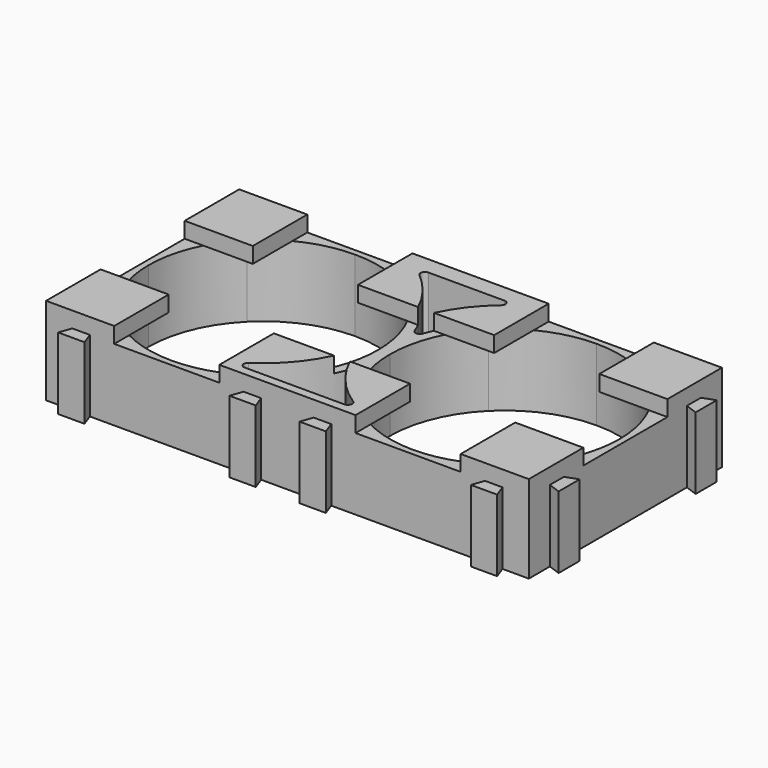
from build123d import *

# Parameters (mm, degrees)
F1_DEPTH = 8.2
F3_DEPTH = 1.8
F5_DEPTH = 8


# Not quite as in the source:
# - a feature names something its author has since deleted; it is built from what else it names


with BuildPart() as f1:
    # F0 (on Top) → F1 (new body)
    with BuildSketch(Plane.XY):
        with BuildLine():
            Line((13.775, 10.775), (13.775, 13.775))
            Line((13.775, 13.775), (10.775, 13.775))
            Line((10.775, 13.775), (11.275, 12.375))
            Line((11.275, 12.375), (8.275, 12.375))
            Line((8.275, 12.375), (8.775, 13.775))
            Line((8.775, 13.775), (0, 13.775))
            Line((0, 13.775), (0, 13.1))
            ThreePointArc((0, 13.1), (9.2630988335, 9.2630988335), (13.1, 0))
            Line((13.1, 0), (13.775, 0))
            Line((13.775, 0), (13.775, 8.775))
            Line((13.775, 8.775), (13.775, 10.775))
        make_face()
        Polygon((15.175, 11.275), (13.775, 10.775), (13.775, 8.775), (15.175, 8.275), align=None)
        Polygon((15.175, -8.275), (13.775, -8.775), (13.775, -10.775), (15.175, -11.275), align=None)
        with BuildLine():
            Line((13.775, -8.775), (13.775, 0))
            Line((13.775, 0), (13.1, 0))
            ThreePointArc((13.1, 0), (12.1028218759, -5.013152964), (9.2630988335, -9.2630988335))
            Line((9.2630988335, -9.2630988335), (13.775, -13.775))
            Line((13.775, -13.775), (13.775, -10.775))
            Line((13.775, -10.775), (13.775, -8.775))
        make_face()
        with BuildLine():
            Line((13.775, -13.775), (9.2630988335, -9.2630988335))
            ThreePointArc((9.2630988335, -9.2630988335), (5.013152964, -12.1028218759), (0, -13.1))
            Line((0, -13.1), (0, -13.775))
            Line((0, -13.775), (8.775, -13.775))
            Line((8.775, -13.775), (10.775, -13.775))
            Line((10.775, -13.775), (13.775, -13.775))
        make_face()
        Polygon((11.275, -15.175), (10.775, -13.775), (8.775, -13.775), (8.275, -15.175), align=None)
        with BuildLine():
            ThreePointArc((0, -13.1), (-9.2630988335, -9.2630988335), (-13.1, 0))
            Line((-13.1, 0), (-13.775, 0))
            Line((-13.775, 0), (-13.775, -8.775))
            Line((-13.775, -8.775), (-12.375, -8.275))
            Line((-12.375, -8.275), (-12.375, -11.275))
            Line((-12.375, -11.275), (-13.775, -10.775))
            Line((-13.775, -10.775), (-13.775, -13.775))
            Line((-13.775, -13.775), (-10.775, -13.775))
            Line((-10.775, -13.775), (-8.775, -13.775))
            Line((-8.775, -13.775), (0, -13.775))
            Line((0, -13.775), (0, -13.1))
        make_face()
        Polygon((-8.275, -15.175), (-8.775, -13.775), (-10.775, -13.775), (-11.275, -15.175), align=None)
        with BuildLine():
            ThreePointArc((-13.1, 0), (-12.1028218759, 5.013152964), (-9.2630988335, 9.2630988335))
            Line((-9.2630988335, 9.2630988335), (-13.775, 13.775))
            Line((-13.775, 13.775), (-13.775, 10.775))
            Line((-13.775, 10.775), (-12.375, 11.275))
            Line((-12.375, 11.275), (-12.375, 8.275))
            Line((-12.375, 8.275), (-13.775, 8.775))
            Line((-13.775, 8.775), (-13.775, 0))
            Line((-13.775, 0), (-13.1, 0))
        make_face()
        with BuildLine():
            Line((0, 13.1), (0, 13.775))
            Line((0, 13.775), (-8.775, 13.775))
            Line((-8.775, 13.775), (-8.275, 12.375))
            Line((-8.275, 12.375), (-9.775, 12.375))
            Line((-9.775, 12.375), (-11.275, 12.375))
            Line((-11.275, 12.375), (-10.775, 13.775))
            Line((-10.775, 13.775), (-13.775, 13.775))
            Line((-13.775, 13.775), (-9.2630988335, 9.2630988335))
            ThreePointArc((-9.2630988335, 9.2630988335), (-5.013152964, 12.1028218759), (0, 13.1))
        make_face()
        with BuildLine():
            ThreePointArc((27.55, -13.1), (18.2869011665, -9.2630988335), (14.45, 0))
            Line((14.45, 0), (13.775, 0))
            Line((13.775, 0), (13.775, -8.775))
            Line((13.775, -8.775), (15.175, -8.275))
            Line((15.175, -8.275), (15.175, -11.275))
            Line((15.175, -11.275), (13.775, -10.775))
            Line((13.775, -10.775), (13.775, -13.775))
            Line((13.775, -13.775), (16.775, -13.775))
            Line((16.775, -13.775), (18.775, -13.775))
            Line((18.775, -13.775), (27.55, -13.775))
            Line((27.55, -13.775), (27.55, -13.1))
        make_face()
        with BuildLine():
            Line((18.2869011665, 9.2630988335), (13.775, 13.775))
            Line((13.775, 13.775), (13.775, 10.775))
            Line((13.775, 10.775), (15.175, 11.275))
            Line((15.175, 11.275), (15.175, 8.275))
            Line((15.175, 8.275), (13.775, 8.775))
            Line((13.775, 8.775), (13.775, 0))
            Line((13.775, 0), (14.45, 0))
            ThreePointArc((14.45, 0), (15.4471781241, 5.013152964), (18.2869011665, 9.2630988335))
        make_face()
        with BuildLine():
            Line((16.775, 13.775), (13.775, 13.775))
            Line((13.775, 13.775), (18.2869011665, 9.2630988335))
            ThreePointArc((18.2869011665, 9.2630988335), (22.536847036, 12.1028218759), (27.55, 13.1))
            Line((27.55, 13.1), (27.55, 13.775))
            Line((27.55, 13.775), (18.775, 13.775))
            Line((18.775, 13.775), (19.275, 12.375))
            Line((19.275, 12.375), (17.775, 12.375))
            Line((17.775, 12.375), (16.275, 12.375))
            Line((16.275, 12.375), (16.775, 13.775))
        make_face()
        with BuildLine():
            Line((27.55, 13.775), (27.55, 13.1))
            ThreePointArc((27.55, 13.1), (36.8130988335, 9.2630988335), (40.65, 0))
            Line((40.65, 0), (41.325, 0))
            Line((41.325, 0), (41.325, 8.775))
            Line((41.325, 8.775), (41.325, 10.775))
            Line((41.325, 10.775), (41.325, 13.775))
            Line((41.325, 13.775), (38.325, 13.775))
            Line((38.325, 13.775), (38.825, 12.375))
            Line((38.825, 12.375), (35.825, 12.375))
            Line((35.825, 12.375), (36.325, 13.775))
            Line((36.325, 13.775), (27.55, 13.775))
        make_face()
        Polygon((41.325, 10.775), (41.325, 8.775), (42.725, 8.275), (42.725, 11.275), align=None)
        Polygon((19.275, -15.175), (18.775, -13.775), (16.775, -13.775), (16.275, -15.175), align=None)
        Polygon((38.325, -13.775), (36.325, -13.775), (35.825, -15.175), (38.825, -15.175), align=None)
        Polygon((42.725, -8.275), (41.325, -8.775), (41.325, -10.775), (42.725, -11.275), align=None)
        with BuildLine():
            Line((41.325, 0), (40.65, 0))
            ThreePointArc((40.65, 0), (39.6528218759, -5.013152964), (36.8130988335, -9.2630988335))
            Line((36.8130988335, -9.2630988335), (41.325, -13.775))
            Line((41.325, -13.775), (41.325, -10.775))
            Line((41.325, -10.775), (41.325, -8.775))
            Line((41.325, -8.775), (41.325, 0))
        make_face()
        with BuildLine():
            ThreePointArc((36.8130988335, -9.2630988335), (32.563152964, -12.1028218759), (27.55, -13.1))
            Line((27.55, -13.1), (27.55, -13.775))
            Line((27.55, -13.775), (36.325, -13.775))
            Line((36.325, -13.775), (38.325, -13.775))
            Line((38.325, -13.775), (41.325, -13.775))
            Line((41.325, -13.775), (36.8130988335, -9.2630988335))
        make_face()
    extrude(amount=F1_DEPTH)

    # F2 (on face) → F3 (join)
    with BuildSketch(Plane.XY.offset(8.2)):
        Polygon((11.275, 12.375), (10.775, 13.775), (8.775, 13.775), (8.275, 12.375), align=None)
        Polygon((-8.775, 13.775), (-10.775, 13.775), (-11.275, 12.375), (-8.275, 12.375), align=None)
        Polygon((-12.375, 11.275), (-13.775, 10.775), (-13.775, 8.775), (-12.375, 8.275), align=None)
        Polygon((-13.775, -8.775), (-13.775, -10.775), (-12.375, -11.275), (-12.375, -8.275), align=None)
        Polygon((18.775, 13.775), (16.775, 13.775), (16.275, 12.375), (19.275, 12.375), align=None)
        Polygon((38.325, 13.775), (36.325, 13.775), (35.825, 12.375), (38.825, 12.375), align=None)
        with BuildLine():
            ThreePointArc((21.55, 11.6451706729), (18.2869011665, 9.2630988335), (15.9048293271, 6))
            Line((15.9048293271, 6), (21.55, 6))
            Line((21.55, 6), (21.55, 11.6451706729))
        make_face()
        with BuildLine():
            ThreePointArc((39.1951706729, 6), (36.8130988335, 9.2630988335), (33.55, 11.6451706729))
            Line((33.55, 11.6451706729), (33.55, 6))
            Line((33.55, 6), (39.1951706729, 6))
        make_face()
        with BuildLine():
            Line((33.55, -6), (33.55, -11.6451706729))
            ThreePointArc((33.55, -11.6451706729), (36.8130988335, -9.2630988335), (39.1951706729, -6))
            Line((39.1951706729, -6), (33.55, -6))
        make_face()
        with BuildLine():
            Line((21.55, -6), (15.9048293271, -6))
            ThreePointArc((15.9048293271, -6), (18.2869011665, -9.2630988335), (21.55, -11.6451706729))
            Line((21.55, -11.6451706729), (21.55, -6))
        make_face()
        with BuildLine():
            Line((-9.2630988335, 9.2630988335), (-6, 6))
            Line((-6, 6), (-6, 11.6451706729))
            ThreePointArc((-6, 11.6451706729), (-7.7239311922, 10.5806846157), (-9.2630988335, 9.2630988335))
        make_face()
        with BuildLine():
            Line((-11.6451706729, 6), (-6, 6))
            Line((-6, 6), (-9.2630988335, 9.2630988335))
            ThreePointArc((-9.2630988335, 9.2630988335), (-10.5806846157, 7.7239311922), (-11.6451706729, 6))
        make_face()
        with BuildLine():
            Line((11.6451706729, -6), (6, -6))
            Line((6, -6), (9.2630988335, -9.2630988335))
            ThreePointArc((9.2630988335, -9.2630988335), (10.5806846157, -7.7239311922), (11.6451706729, -6))
        make_face()
        with BuildLine():
            Line((9.2630988335, -9.2630988335), (6, -6))
            Line((6, -6), (6, -11.6451706729))
            ThreePointArc((6, -11.6451706729), (7.7239311922, -10.5806846157), (9.2630988335, -9.2630988335))
        make_face()
        with BuildLine():
            Line((6, 11.6451706729), (6, 6))
            Line((6, 6), (9.2630988335, 9.2630988335))
            ThreePointArc((9.2630988335, 9.2630988335), (7.7239311922, 10.5806846157), (6, 11.6451706729))
        make_face()
        with BuildLine():
            Line((9.2630988335, 9.2630988335), (6, 6))
            Line((6, 6), (11.6451706729, 6))
            ThreePointArc((11.6451706729, 6), (10.5806846157, 7.7239311922), (9.2630988335, 9.2630988335))
        make_face()
        with BuildLine():
            Line((-9.2630988335, -9.2630988335), (-6, -6))
            Line((-6, -6), (-11.6451706729, -6))
            ThreePointArc((-11.6451706729, -6), (-10.5806846157, -7.7239311922), (-9.2630988335, -9.2630988335))
        make_face()
        with BuildLine():
            Line((-6, -11.6451706729), (-6, -6))
            Line((-6, -6), (-9.2630988335, -9.2630988335))
            ThreePointArc((-9.2630988335, -9.2630988335), (-7.7239311922, -10.5806846157), (-6, -11.6451706729))
        make_face()
        with BuildLine():
            Line((13.775, -13.775), (9.2630988335, -9.2630988335))
            ThreePointArc((9.2630988335, -9.2630988335), (7.7239311922, -10.5806846157), (6, -11.6451706729))
            Line((6, -11.6451706729), (6, -13.775))
            Line((6, -13.775), (8.775, -13.775))
            Line((8.775, -13.775), (10.775, -13.775))
            Line((10.775, -13.775), (13.775, -13.775))
        make_face()
        with BuildLine():
            ThreePointArc((11.6451706729, -6), (10.5806846157, -7.7239311922), (9.2630988335, -9.2630988335))
            Line((9.2630988335, -9.2630988335), (13.775, -13.775))
            Line((13.775, -13.775), (13.775, -6))
            Line((13.775, -6), (11.6451706729, -6))
        make_face()
        with BuildLine():
            ThreePointArc((-11.6451706729, 6), (-10.5806846157, 7.7239311922), (-9.2630988335, 9.2630988335))
            Line((-9.2630988335, 9.2630988335), (-13.775, 13.775))
            Line((-13.775, 13.775), (-13.775, 10.775))
            Line((-13.775, 10.775), (-12.375, 11.275))
            Line((-12.375, 11.275), (-12.375, 8.275))
            Line((-12.375, 8.275), (-13.775, 8.775))
            Line((-13.775, 8.775), (-13.775, 6))
            Line((-13.775, 6), (-11.6451706729, 6))
        make_face()
        with BuildLine():
            Line((-13.775, 13.775), (-9.2630988335, 9.2630988335))
            ThreePointArc((-9.2630988335, 9.2630988335), (-7.7239311922, 10.5806846157), (-6, 11.6451706729))
            Line((-6, 11.6451706729), (-6, 13.775))
            Line((-6, 13.775), (-8.775, 13.775))
            Line((-8.775, 13.775), (-8.275, 12.375))
            Line((-8.275, 12.375), (-11.275, 12.375))
            Line((-11.275, 12.375), (-10.775, 13.775))
            Line((-10.775, 13.775), (-13.775, 13.775))
        make_face()
        with BuildLine():
            ThreePointArc((6, 11.6451706729), (7.7239311922, 10.5806846157), (9.2630988335, 9.2630988335))
            Line((9.2630988335, 9.2630988335), (13.775, 13.775))
            Line((13.775, 13.775), (10.775, 13.775))
            Line((10.775, 13.775), (11.275, 12.375))
            Line((11.275, 12.375), (8.275, 12.375))
            Line((8.275, 12.375), (8.775, 13.775))
            Line((8.775, 13.775), (6, 13.775))
            Line((6, 13.775), (6, 11.6451706729))
        make_face()
        with BuildLine():
            Line((13.775, 13.775), (9.2630988335, 9.2630988335))
            ThreePointArc((9.2630988335, 9.2630988335), (10.5806846157, 7.7239311922), (11.6451706729, 6))
            Line((11.6451706729, 6), (13.775, 6))
            Line((13.775, 6), (13.775, 13.775))
        make_face()
        with BuildLine():
            Line((-13.775, -13.775), (-9.2630988335, -9.2630988335))
            ThreePointArc((-9.2630988335, -9.2630988335), (-10.5806846157, -7.7239311922), (-11.6451706729, -6))
            Line((-11.6451706729, -6), (-13.775, -6))
            Line((-13.775, -6), (-13.775, -8.775))
            Line((-13.775, -8.775), (-12.375, -8.275))
            Line((-12.375, -8.275), (-12.375, -11.275))
            Line((-12.375, -11.275), (-13.775, -10.775))
            Line((-13.775, -10.775), (-13.775, -13.775))
        make_face()
        with BuildLine():
            ThreePointArc((-6, -11.6451706729), (-7.7239311922, -10.5806846157), (-9.2630988335, -9.2630988335))
            Line((-9.2630988335, -9.2630988335), (-13.775, -13.775))
            Line((-13.775, -13.775), (-10.775, -13.775))
            Line((-10.775, -13.775), (-8.775, -13.775))
            Line((-8.775, -13.775), (-6, -13.775))
            Line((-6, -13.775), (-6, -11.6451706729))
        make_face()
        with BuildLine():
            Line((16.775, 13.775), (13.775, 13.775))
            Line((13.775, 13.775), (13.775, 6))
            Line((13.775, 6), (15.9048293271, 6))
            ThreePointArc((15.9048293271, 6), (18.2869011665, 9.2630988335), (21.55, 11.6451706729))
            Line((21.55, 11.6451706729), (21.55, 13.775))
            Line((21.55, 13.775), (18.775, 13.775))
            Line((18.775, 13.775), (19.275, 12.375))
            Line((19.275, 12.375), (16.275, 12.375))
            Line((16.275, 12.375), (16.775, 13.775))
        make_face()
        with BuildLine():
            Line((33.55, 13.775), (33.55, 11.6451706729))
            ThreePointArc((33.55, 11.6451706729), (36.8130988335, 9.2630988335), (39.1951706729, 6))
            Line((39.1951706729, 6), (41.325, 6))
            Line((41.325, 6), (41.325, 8.775))
            Line((41.325, 8.775), (41.325, 10.775))
            Line((41.325, 10.775), (41.325, 13.775))
            Line((41.325, 13.775), (38.325, 13.775))
            Line((38.325, 13.775), (38.825, 12.375))
            Line((38.825, 12.375), (35.825, 12.375))
            Line((35.825, 12.375), (36.325, 13.775))
            Line((36.325, 13.775), (33.55, 13.775))
        make_face()
        with BuildLine():
            ThreePointArc((39.1951706729, -6), (36.8130988335, -9.2630988335), (33.55, -11.6451706729))
            Line((33.55, -11.6451706729), (33.55, -13.775))
            Line((33.55, -13.775), (36.325, -13.775))
            Line((36.325, -13.775), (38.325, -13.775))
            Line((38.325, -13.775), (41.325, -13.775))
            Line((41.325, -13.775), (41.325, -10.775))
            Line((41.325, -10.775), (41.325, -8.775))
            Line((41.325, -8.775), (41.325, -6))
            Line((41.325, -6), (39.1951706729, -6))
        make_face()
        with BuildLine():
            Line((13.775, -6), (13.775, -13.775))
            Line((13.775, -13.775), (16.775, -13.775))
            Line((16.775, -13.775), (18.775, -13.775))
            Line((18.775, -13.775), (21.55, -13.775))
            Line((21.55, -13.775), (21.55, -11.6451706729))
            ThreePointArc((21.55, -11.6451706729), (18.2869011665, -9.2630988335), (15.9048293271, -6))
            Line((15.9048293271, -6), (13.775, -6))
        make_face()
    extrude(amount=F3_DEPTH)

    # F4 (on face) → F5 (cut)
    with BuildSketch(Plane.XY.offset(10)):
        with BuildLine():
            ThreePointArc((14.275, -5.1321900783), (13.6863115297, -5.6242615723), (13.3064625791, -4.9576258059))
            ThreePointArc((13.3064625791, -4.9576258059), (11.1089149295, -8.8448860417), (7.8128161467, -11.8574830321))
            ThreePointArc((7.8128161467, -11.8574830321), (8.3250338925, -11.8348014024), (8.587915368, -12.275))
            ThreePointArc((8.587915368, -12.275), (8.4414687586, -12.6285533906), (8.087915368, -12.775))
            Line((8.087915368, -12.775), (19.462084632, -12.775))
            ThreePointArc((19.462084632, -12.775), (18.9831490904, -12.1314007418), (19.737183786, -11.8574829878))
            ThreePointArc((19.737183786, -11.8574829878), (16.4410850319, -8.8448859932), (14.2435374058, -4.9576257653))
            ThreePointArc((14.2435374058, -4.9576257653), (14.2670714902, -5.0435015867), (14.275, -5.1321900783))
        make_face()
        with BuildLine():
            ThreePointArc((8.587915368, -12.275), (8.3250338925, -11.8348014024), (7.8128161467, -11.8574830321))
            ThreePointArc((7.8128161467, -11.8574830321), (7.6089798379, -12.4185992968), (8.087915368, -12.775))
            ThreePointArc((8.087915368, -12.775), (8.4414687586, -12.6285533906), (8.587915368, -12.275))
        make_face()
        with BuildLine():
            ThreePointArc((19.962084632, -12.275), (19.9022832105, -12.03788144), (19.737183786, -11.8574829878))
            ThreePointArc((19.737183786, -11.8574829878), (18.9831490904, -12.1314007418), (19.462084632, -12.775))
            ThreePointArc((19.462084632, -12.775), (19.8156380226, -12.6285533906), (19.962084632, -12.275))
        make_face()
        with BuildLine():
            ThreePointArc((14.275, 5.1321900783), (13.6863115269, 5.6242615719), (13.306462581, 4.9576258007))
            ThreePointArc((13.306462581, 4.9576258007), (13.7749999905, 4.6321900783), (14.2435374124, 4.957625783))
            ThreePointArc((14.2435374124, 4.957625783), (14.2670714919, 5.0435015959), (14.275, 5.1321900783))
        make_face()
        with BuildLine():
            ThreePointArc((9.1112733402, 10.8914965969), (11.2595338629, 8.6523347826), (12.8701204346, 6))
            Line((12.8701204346, 6), (14.6798795654, 6))
            ThreePointArc((14.6798795654, 6), (16.2904661313, 8.6523347751), (18.4387266452, 10.8914965847))
            ThreePointArc((18.4387266452, 10.8914965847), (17.6479328663, 11.1043420199), (18.1179071781, 11.775))
            Line((18.1179071781, 11.775), (9.4320928219, 11.775))
            ThreePointArc((9.4320928219, 11.775), (9.7856462124, 11.6285533906), (9.9320928219, 11.275))
            ThreePointArc((9.9320928219, 11.275), (9.6437414211, 10.8220045581), (9.1112733402, 10.8914965969))
        make_face()
        with BuildLine():
            ThreePointArc((9.4320928219, 11.775), (8.9621185132, 11.445657989), (9.1112733402, 10.8914965969))
            ThreePointArc((9.1112733402, 10.8914965969), (9.6437414211, 10.8220045581), (9.9320928219, 11.275))
            ThreePointArc((9.9320928219, 11.275), (9.7856462124, 11.6285533906), (9.4320928219, 11.775))
        make_face()
        with BuildLine():
            ThreePointArc((18.1179071781, 11.775), (17.6479328663, 11.1043420199), (18.4387266452, 10.8914965847))
            ThreePointArc((18.4387266452, 10.8914965847), (18.570902616, 11.0633513921), (18.6179071781, 11.275))
            ThreePointArc((18.6179071781, 11.275), (18.4714605687, 11.6285533906), (18.1179071781, 11.775))
        make_face()
        with BuildLine():
            ThreePointArc((12.8701204346, 6), (13.0986644581, 5.4831550602), (13.306462581, 4.9576258007))
            ThreePointArc((13.306462581, 4.9576258007), (13.6863115269, 5.6242615719), (14.275, 5.1321900783))
            ThreePointArc((14.275, 5.1321900783), (14.2670714919, 5.0435015959), (14.2435374124, 4.957625783))
            ThreePointArc((14.2435374124, 4.957625783), (14.4513355383, 5.4831550515), (14.6798795654, 6))
            Line((14.6798795654, 6), (12.8701204346, 6))
        make_face()
        with BuildLine():
            ThreePointArc((14.2435374058, -4.9576257653), (13.7749999783, -4.6321900783), (13.3064625791, -4.9576258059))
            ThreePointArc((13.3064625791, -4.9576258059), (13.6863115297, -5.6242615723), (14.275, -5.1321900783))
            ThreePointArc((14.275, -5.1321900783), (14.2670714902, -5.0435015867), (14.2435374058, -4.9576257653))
        make_face()
    extrude(amount=-F5_DEPTH, mode=Mode.SUBTRACT)


solid = f1.part
